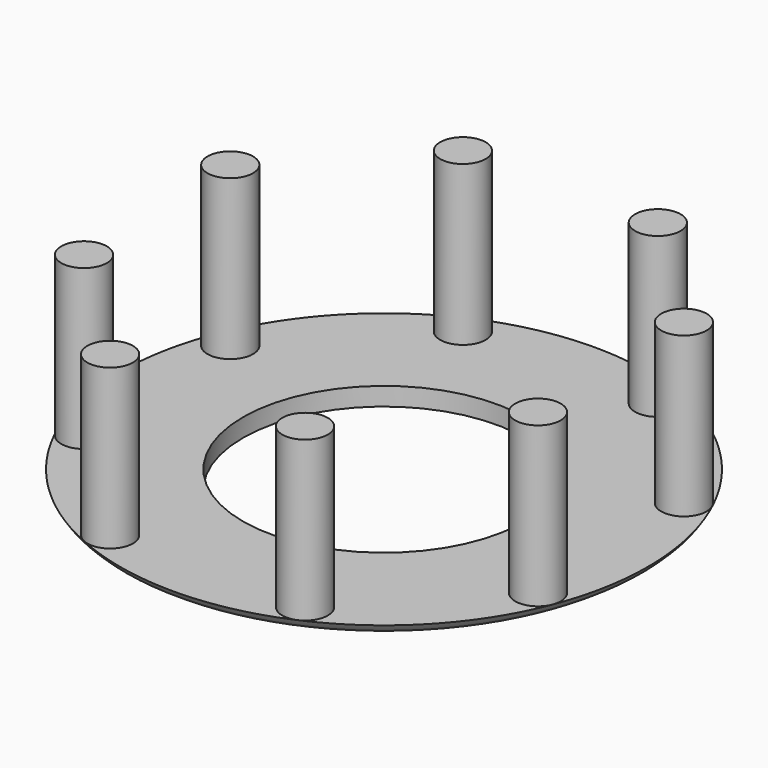
from build123d import *

# Parameters (mm, degrees)
F0_W     = 38.1
F0_H     = 10.16
F2_R     = 12.7
F3_DEPTH = 88.9
F4_DEPTH = 88.9


# Not quite as in the source:
# - a feature names something its author has since deleted; it is built from what else it names


with BuildPart() as f1:
    # F0 (on Front) → F1 (revolve)
    with BuildSketch(Plane.XZ):
        with BuildLine():
            add(Edge.make_bspline(
                [(-147.2955053902, 10.16), (-143.5447688246, 2.570837969), (-131.58254077, 0), (-116.84, 0)],
                knots=[0, 0, 0, 0, 32.1055043345, 32.1055043345, 32.1055043345, 32.1055043345], degree=3))
            Line((-116.84, 0), (-116.84, 10.16))
            Line((-116.84, 10.16), (-147.2955053902, 10.16))
        make_face()
        with Locations((-97.79, 5.08)):
            Rectangle(F0_W, F0_H)
    revolve(axis=Axis((0, 0, 13.0290351808), (0, 0, -1)))

    # F2 (on face) → F3 (join)
    with BuildSketch(Plane.XY.offset(10.16)):
        with Locations((-54.3942935765, 123.0764985085)):
            Circle(F2_R)
        with Locations((54.3942935765, 123.0764985085)):
            Circle(F2_R)
        with Locations((121.978003574, 56.8147908631)):
            Circle(F2_R)
        with Locations((125.2771361136, -49.1679397622)):
            Circle(F2_R)
        with Locations((54.3942935765, -123.0764985085)):
            Circle(F2_R)
        with Locations((-54.3942935765, -123.0764985085)):
            Circle(F2_R)
        with Locations((-121.9781520783, -56.8146452636)):
            Circle(F2_R)
    extrude(amount=F3_DEPTH)

    # F2 (on face) → F4 (join)
    with BuildSketch(Plane.XY.offset(10.16)):
        with Locations((-125.2057118813, 49.2424128206)):
            Circle(F2_R)
    extrude(amount=F4_DEPTH)


solid = f1.part
